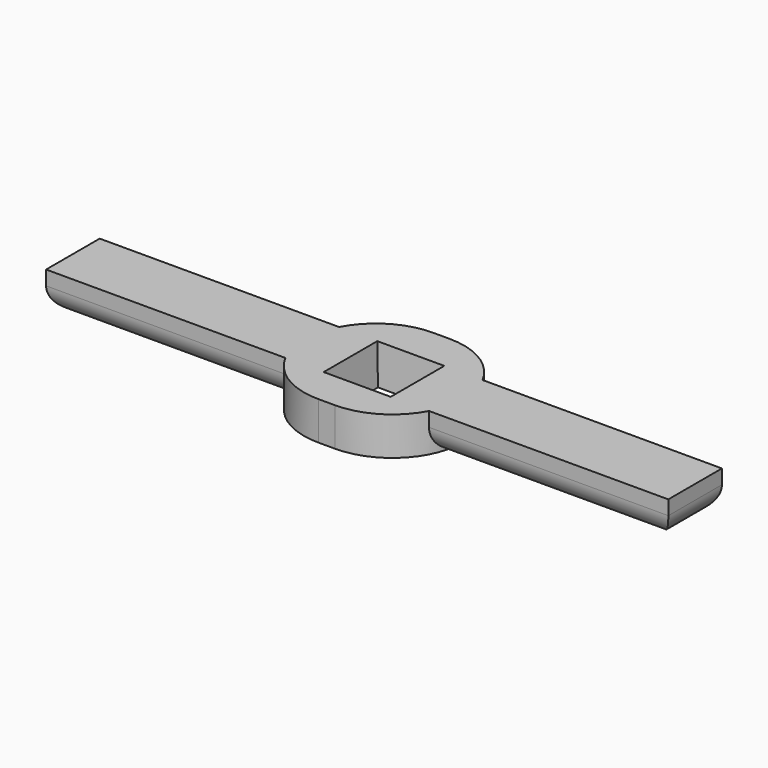
from build123d import *

# Parameters (mm, degrees)
F0_W        = 15
F0_H        = 15
F0_W_2      = 7
F0_H_2      = 7
F1_DEPTH    = 4
F2_W        = 7
F2_H        = 7
F3_DEPTH    = 4
F3_TAPER    = 5
F4_W        = 7
F4_H        = 4
F5_DEPTH    = 25
F6_W        = 7
F6_H        = 4
F7_DEPTH    = 25
F8_T1_DEPTH = 37.1662479036
F9_R        = 2.5


# Not quite as in the source:
# - a fillet or chamfer that OpenCascade refuses, or shapes differently, is made with other operations: its cross-section is extruded or revolved along the edge and cut away or added


with BuildPart() as f1:
    # F0 (on Top) → F1 (new body)
    with BuildSketch(Plane.XY):
        Rectangle(F0_W, F0_H)
        Rectangle(F0_W_2, F0_H_2, mode=Mode.SUBTRACT)
        Rectangle(F0_W_2, F0_H_2)
    extrude(amount=F1_DEPTH)

    # F2 (on face) → F3 (cut)
    with BuildSketch(Plane.XY.offset(4)):
        Rectangle(F2_W, F2_H)
    extrude(amount=-F3_DEPTH, taper=F3_TAPER, mode=Mode.SUBTRACT)

    # F4 (on face) → F5 (join)
    with BuildSketch(Plane.YZ.offset(7.5)):
        with Locations((0, 2)):
            Rectangle(F4_W, F4_H)
    extrude(amount=F5_DEPTH)

    # F6 (on face) → F7 (join)
    with BuildSketch(Plane(origin=(-7.5, 0, 0), x_dir=(0, -1, 0), z_dir=(-1, 0, 0))):
        with Locations((0, 2)):
            Rectangle(F6_W, F6_H)
    extrude(amount=F7_DEPTH)

    # F8: fillet of radius 7.5 on 4 edges, made by hand

    # F8_s2 → F8_t1 (cut)
    with BuildSketch(Plane.XY.offset(-16.5831239518)):
        with BuildLine():
            ThreePointArc((-0.8667504193, 7.5), (-4.7397337655, 6.4226162893), (-7.5, 3.5))
            Line((-7.5, 3.5), (-7.5, 7.5))
            Line((-7.5, 7.5), (-0.8667504193, 7.5))
        make_face()
        with BuildLine():
            ThreePointArc((7.5, 3.5), (4.7397337655, 6.4226162893), (0.8667504193, 7.5))
            Line((0.8667504193, 7.5), (7.5, 7.5))
            Line((7.5, 7.5), (7.5, 3.5))
        make_face()
        with BuildLine():
            ThreePointArc((7.5, -3.5), (4.7397337655, -6.4226162893), (0.8667504193, -7.5))
            Line((0.8667504193, -7.5), (7.5, -7.5))
            Line((7.5, -7.5), (7.5, -3.5))
        make_face()
        with BuildLine():
            ThreePointArc((-0.8667504193, -7.5), (-4.7397337655, -6.4226162893), (-7.5, -3.5))
            Line((-7.5, -3.5), (-7.5, -7.5))
            Line((-7.5, -7.5), (-0.8667504193, -7.5))
        make_face()
    extrude(amount=F8_T1_DEPTH, mode=Mode.SUBTRACT)

    # F9
    f9_edges = [f1.edges().sort_by_distance(p)[0] for p in [
        (-32.5, 0, 0),
        (-20, -3.5, 0),
        (-20, 3.5, 0),
        (20, 3.5, 0),
        (32.5, 0, 0),
        (20, -3.5, 0),
    ]]
    fillet(f9_edges, radius=F9_R)


solid = f1.part
